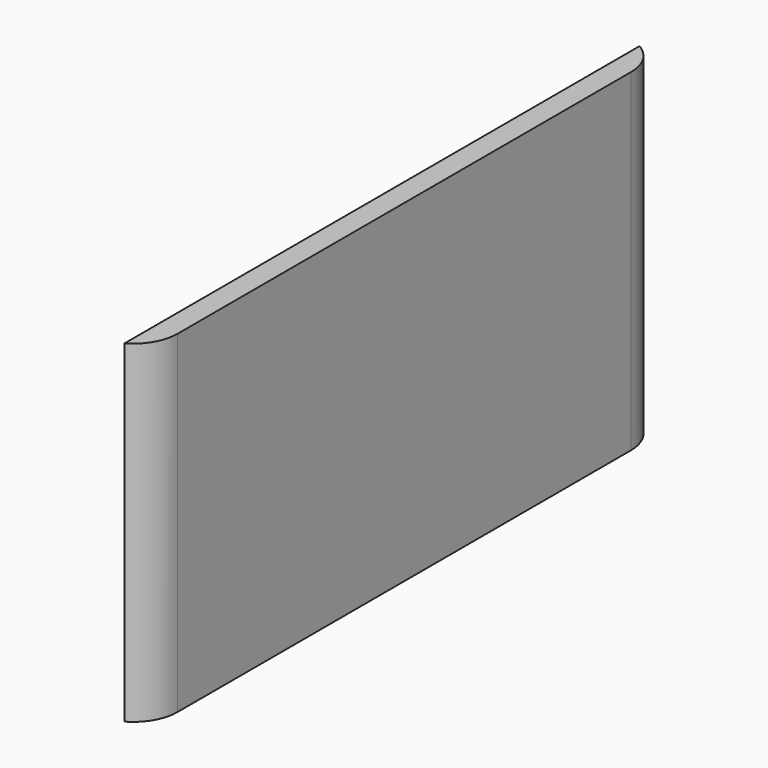
from build123d import *

# Parameters (mm, degrees)
F0_W        = 2.54
F0_H        = 38.1
F1_DEPTH    = 73.66
F2_T1_DEPTH = 60.0970452561


# Not quite as in the source:
# - a fillet or chamfer that OpenCascade refuses, or shapes differently, is made with other operations: its cross-section is extruded or revolved along the edge and cut away or added


with BuildPart() as f1:
    # F0 (on Front) → F1 (new body)
    with BuildSketch(Plane.XZ):
        with Locations((1.27, 19.05)):
            Rectangle(F0_W, F0_H)
    extrude(amount=F1_DEPTH)

    # F2: fillet of radius 5.08 on 2 edges, made by hand

    # F2_s2 → F2_t1 (cut)
    with BuildSketch(Plane.XY.offset(-10.9985226281)):
        with BuildLine():
            ThreePointArc((2.54, -69.2605909488), (1.8594090512, -71.8005909488), (0, -73.66))
            Line((0, -73.66), (2.54, -73.66))
            Line((2.54, -73.66), (2.54, -69.2605909488))
        make_face()
        with BuildLine():
            ThreePointArc((2.54, -4.3994090512), (1.8594090512, -1.8594090512), (0, 0))
            Line((0, 0), (2.54, 0))
            Line((2.54, 0), (2.54, -4.3994090512))
        make_face()
    extrude(amount=F2_T1_DEPTH, mode=Mode.SUBTRACT)


solid = f1.part
